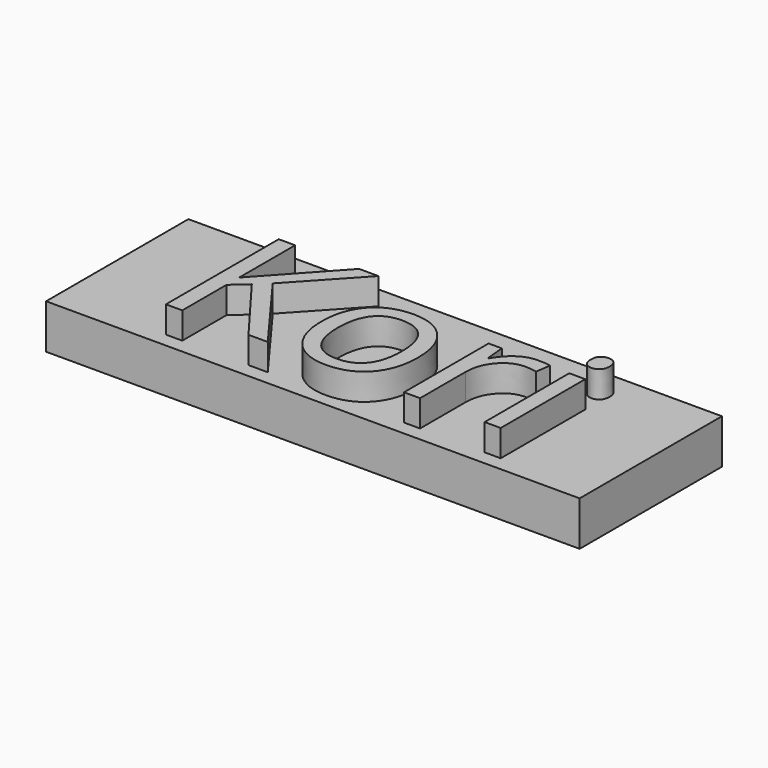
from build123d import *

# Parameters (mm, degrees)
F0_W         = 60
F0_H         = 20
F1_DEPTH     = 5
F2_TEXT_SIZE = 22.2106541732
F3_DEPTH     = 3


# Not quite as in the source:
# - Text() gives the source's letters only with a copy of the font that has no kerning and outlines rounded to 1/6400 em; it was checked with that copy


with BuildPart() as f1:
    # F0 (on Top) → F1 (new body)
    with BuildSketch(Plane.XY):
        Rectangle(F0_W, F0_H)
    extrude(amount=F1_DEPTH)

    # F2 (on face) → F3 (join)
    with BuildSketch(Plane.XY.offset(5)):
        with Locations((-20, -8.3800504646)):
            Text('Kori', F2_TEXT_SIZE, font='Open Sans', text_align=(TextAlign.LEFT, TextAlign.BOTTOM))
    extrude(amount=F3_DEPTH)


solid = f1.part
